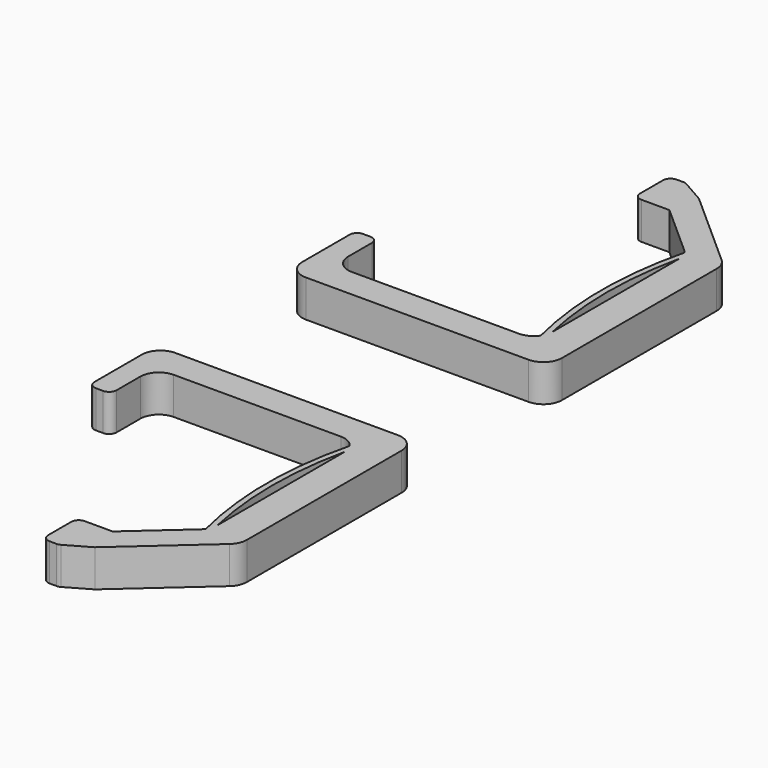
from build123d import *

# Parameters (mm, degrees)
F1_DEPTH = 10
F2_R     = 2


with BuildPart() as f1:
    # F0 (on Top) → F1 (new body)
    with BuildSketch(Plane.XY):
        with BuildLine():
            Line((0, 5), (0, 13))
            ThreePointArc((0, 13), (-0.5857864376, 14.4142135624), (-2, 15))
            Line((-2, 15), (-4, 15))
            ThreePointArc((-4, 15), (-5.4142135624, 14.4142135624), (-6, 13))
            Line((-6, 13), (-6, -3))
            ThreePointArc((-6, -3), (-4.5355339059, -6.5355339059), (-1, -8))
            Line((-1, -8), (59, -8))
            ThreePointArc((59, -8), (62.5355339059, -6.5355339059), (64, -3))
            Line((64, -3), (64, 49.1177613581))
            ThreePointArc((64, 49.1177613581), (63.5617552688, 51.164805292), (62.3238444529, 52.8530067386))
            Line((62.3238444529, 52.8530067386), (41.117766383, 71.7234416849))
            Line((41.117766383, 71.7234416849), (34.4277384529, 75.5467076555))
            Line((34.4277384529, 75.5467076555), (32, 75.5467076555))
            ThreePointArc((32, 75.5467076555), (30.5857864376, 74.9609212178), (30, 73.5467076555))
            Line((30, 73.5467076555), (30, 71.4909657836))
            Line((30, 71.4909657836), (30, 66.5854863102))
            Line((30, 66.5854863102), (30, 65.75772506))
            ThreePointArc((30, 65.75772506), (30.5857864376, 64.3435114976), (32, 63.75772506))
            Line((32, 63.75772506), (33.0982006717, 63.75772506))
            Line((33.0982006717, 63.75772506), (39.5394453007, 63.75772506))
            Line((39.5394453007, 63.75772506), (53.3238444529, 51.4915433258))
            ThreePointArc((53.3238444529, 51.4915433258), (53.7532179323, 51.0598347094), (54.1269336048, 50.5791367685))
            ThreePointArc((54.1269336048, 50.5791367685), (51.143371317, 26.3781489726), (54.1269336048, 2.1771611768))
            ThreePointArc((54.1269336048, 2.1771611768), (52.333002988, 0.5776593236), (50, 0))
            Line((50, 0), (5, 0))
            ThreePointArc((5, 0), (1.4644660941, 1.4644660941), (0, 5))
        make_face()
        with BuildLine():
            Line((55, 47.7562979452), (55, 5))
            ThreePointArc((55, 5), (52.643371317, 26.3781489726), (55, 47.7562979452))
        make_face(mode=Mode.SUBTRACT)
    extrude(amount=F1_DEPTH)

    # F2
    f2_edges = [f1.edges().sort_by_distance(p)[0] for p in [
        (34.427738, 75.546708, 5),
    ]]
    fillet(f2_edges, radius=F2_R)


with BuildPart() as f4_1:
    # F4: instance of F1
    add(f1.part.mirror(Plane.XZ.offset(30)))


solid = Compound([f1.part, f4_1.part])
